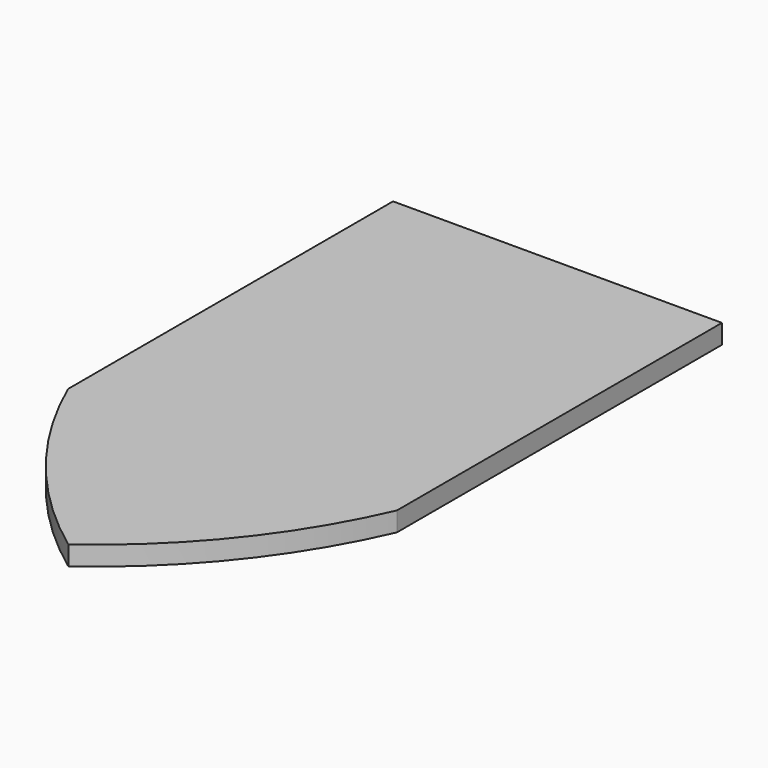
from build123d import *

# Parameters (mm, degrees)
F1_DEPTH = 3.175


# Not quite as in the source:
# - a length typed as a fraction of an inch, garbled in the dataset ("3 / 203.2 mm" for 3/8 in), is restored


with BuildPart() as f1:
    # F0 (on Top) → F1 (new body)
    with BuildSketch(Plane.XY):
        with BuildLine():
            Line((30.8428571429, 51.7197510952), (-23.1321428571, 51.7197510952))
            Line((-23.1321428571, 51.7197510952), (-23.1321428571, -14.9552489048))
            ThreePointArc((-23.1321428571, -14.9552489048), (-11.8746654703, -33.5821135274), (3.8553571429, -48.6239641905))
            ThreePointArc((3.8553571429, -48.6239641905), (19.5853799846, -33.5821137106), (30.8428571429, -14.9552489048))
            Line((30.8428571429, -14.9552489048), (30.8428571429, 51.7197510952))
        make_face()
    extrude(amount=F1_DEPTH)


solid = f1.part
